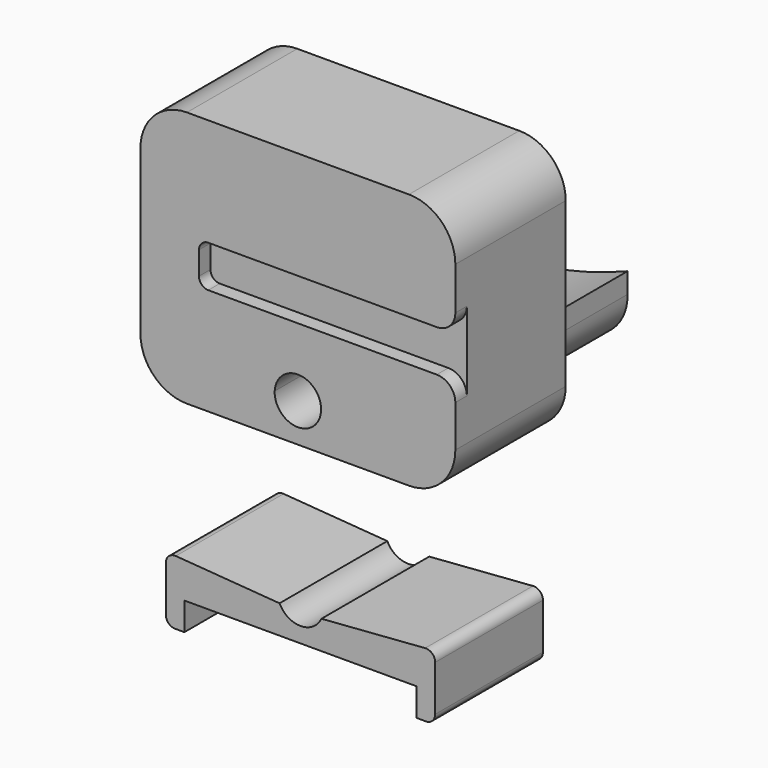
from build123d import *
from build123d import SkipClean  # not in build123d's __all__

# Parameters (mm, degrees)
F1_DEPTH  = 14.85
F2_DEPTH  = 13.3
F3_START  = 4
F3_DEPTH  = 9.3
F4_DEPTH  = 4
F5_START  = 4
F5_DEPTH  = 10.85
F6_R      = 1
F8_DEPTH  = 14.5
F9_DEPTH  = 3
F10_DEPTH = 2
F12_DEPTH = 14.5


with BuildPart() as f1:
    # F0 (on Front) → F1 (new body)
    with BuildSketch(Plane.XZ):
        with BuildLine():
            Line((11.95, 13.8), (-11.95, 13.8))
            ThreePointArc((-11.95, 13.8), (-15.4855339059, 12.3355339059), (-16.95, 8.8))
            Line((-16.95, 8.8), (-16.95, -5.8895261027))
            ThreePointArc((-16.95, -5.8895261027), (-9.8804541895, -8.3334638669), (-2.4972846772, -9.5335129141))
            ThreePointArc((-2.4972846772, -9.5335129141), (0.0448690015, -7.1504026779), (2.4998564985, -9.6232140564))
            ThreePointArc((2.4998564985, -9.6232140564), (9.8559923461, -8.7028657635), (16.95, -6.55))
            Line((16.95, -6.55), (16.95, -4.3))
            ThreePointArc((16.95, -4.3), (16.3642135624, -2.8857864376), (14.95, -2.3))
            Line((14.95, -2.3), (4.4395945761, -2.3))
            ThreePointArc((4.4395945761, -2.3), (0, -5), (-4.4395945761, -2.3))
            Line((-4.4395945761, -2.3), (-10.65, -2.3))
            Line((-10.65, -2.3), (-10.65, 2.2))
            Line((-10.65, 2.2), (-4.4899888641, 2.2))
            ThreePointArc((-4.4899888641, 2.2), (0, 5), (4.4899888641, 2.2))
            Line((4.4899888641, 2.2), (14.95, 2.2))
            ThreePointArc((14.95, 2.2), (16.3642135624, 2.7857864376), (16.95, 4.2))
            Line((16.95, 4.2), (16.95, 8.8))
            ThreePointArc((16.95, 8.8), (15.4855339059, 12.3355339059), (11.95, 13.8))
        make_face()
        with BuildLine():
            ThreePointArc((-2.4972846772, -9.5335129141), (-9.8804541895, -8.3334638669), (-16.95, -5.8895261027))
            Line((-16.95, -5.8895261027), (-16.95, -8.8))
            ThreePointArc((-16.95, -8.8), (-15.4855339059, -12.3355339059), (-11.95, -13.8))
            Line((-11.95, -13.8), (11.95, -13.8))
            ThreePointArc((11.95, -13.8), (15.4855339059, -12.3355339059), (16.95, -8.8))
            Line((16.95, -8.8), (16.95, -6.55))
            ThreePointArc((16.95, -6.55), (9.8559923461, -8.7028657635), (2.4998564985, -9.6232140564))
            ThreePointArc((2.4998564985, -9.6232140564), (2.4999641244, -9.636606836), (2.5, -9.65))
            ThreePointArc((2.5, -9.65), (-0.0582593644, -12.1493210771), (-2.4972846772, -9.5335129141))
        make_face()
    extrude(amount=F1_DEPTH)

    # F0 (on Front) → F2 (join)
    with BuildSketch(Plane.XZ):
        with BuildLine():
            ThreePointArc((-4.4395945761, -2.3), (-4.9996865006, -0.0559901426), (-4.4899888641, 2.2))
            Line((-4.4899888641, 2.2), (-10.65, 2.2))
            Line((-10.65, 2.2), (-10.65, -2.3))
            Line((-10.65, -2.3), (-4.4395945761, -2.3))
        make_face()
        with BuildLine():
            ThreePointArc((5, 0), (4.8708286934, 1.1291713066), (4.4899888641, 2.2))
            Line((4.4899888641, 2.2), (-4.4899888641, 2.2))
            ThreePointArc((-4.4899888641, 2.2), (-4.9996865006, -0.0559901426), (-4.4395945761, -2.3))
            Line((-4.4395945761, -2.3), (4.4395945761, -2.3))
            ThreePointArc((4.4395945761, -2.3), (4.8578788005, -1.1836441863), (5, 0))
        make_face()
        with BuildLine():
            Line((16.95, 2.2), (16.95, 4.2))
            ThreePointArc((16.95, 4.2), (16.3642135624, 2.7857864376), (14.95, 2.2))
            Line((14.95, 2.2), (4.4899888641, 2.2))
            ThreePointArc((4.4899888641, 2.2), (4.8708286934, 1.1291713066), (5, 0))
            ThreePointArc((5, 0), (4.8578788005, -1.1836441863), (4.4395945761, -2.3))
            Line((4.4395945761, -2.3), (14.95, -2.3))
            ThreePointArc((14.95, -2.3), (16.3642135624, -2.8857864376), (16.95, -4.3))
            Line((16.95, -4.3), (16.95, -2.3))
            Line((16.95, -2.3), (16.95, 2.2))
        make_face()
    extrude(amount=F2_DEPTH)

    # F0 (on Front) → F3 (join)
    with BuildSketch(Plane.XZ.offset(F3_START)):
        with BuildLine():
            Line((-4.4899888641, 2.2), (4.4899888641, 2.2))
            ThreePointArc((4.4899888641, 2.2), (0, 5), (-4.4899888641, 2.2))
        make_face()
        with BuildLine():
            Line((4.4395945761, -2.3), (-4.4395945761, -2.3))
            ThreePointArc((-4.4395945761, -2.3), (0, -5), (4.4395945761, -2.3))
        make_face()
        with BuildLine():
            ThreePointArc((5, 0), (4.8708286934, 1.1291713066), (4.4899888641, 2.2))
            Line((4.4899888641, 2.2), (-4.4899888641, 2.2))
            ThreePointArc((-4.4899888641, 2.2), (-4.9996865006, -0.0559901426), (-4.4395945761, -2.3))
            Line((-4.4395945761, -2.3), (4.4395945761, -2.3))
            ThreePointArc((4.4395945761, -2.3), (4.8578788005, -1.1836441863), (5, 0))
        make_face()
    extrude(amount=F3_DEPTH)

    # F0 (on Front) → F4 (cut)
    with BuildSketch(Plane.XZ):
        with BuildLine():
            ThreePointArc((5, 0), (4.8708286934, 1.1291713066), (4.4899888641, 2.2))
            Line((4.4899888641, 2.2), (-4.4899888641, 2.2))
            ThreePointArc((-4.4899888641, 2.2), (-4.9996865006, -0.0559901426), (-4.4395945761, -2.3))
            Line((-4.4395945761, -2.3), (4.4395945761, -2.3))
            ThreePointArc((4.4395945761, -2.3), (4.8578788005, -1.1836441863), (5, 0))
        make_face()
    with SkipClean():  # cleaning this boolean's faces spoils the solid; the shape is the same uncleaned
        extrude(amount=F4_DEPTH, mode=Mode.SUBTRACT)

    # F0 (on Front) → F5 (join)
    with BuildSketch(Plane.XZ.offset(F5_START)):
        with BuildLine():
            Line((-4.4899888641, 2.2), (4.4899888641, 2.2))
            ThreePointArc((4.4899888641, 2.2), (0, 5), (-4.4899888641, 2.2))
        make_face()
        with BuildLine():
            Line((4.4395945761, -2.3), (-4.4395945761, -2.3))
            ThreePointArc((-4.4395945761, -2.3), (0, -5), (4.4395945761, -2.3))
        make_face()
    with SkipClean():  # cleaning this boolean's faces spoils the solid; the shape is the same uncleaned
        extrude(amount=F5_DEPTH)

    # F6
    f6_edges = [f1.edges().sort_by_distance(p)[0] for p in [
        (-10.65, -14.075, 2.2),
        (-10.65, -14.075, -2.3),
    ]]
    fillet(f6_edges, radius=F6_R)


with BuildPart() as f8:
    # F7 (on Front) → F8 (new body)
    with BuildSketch(Plane.XZ):
        with BuildLine():
            ThreePointArc((-21.773402003, -7.6886942186), (-20.308935909, -11.2242281245), (-16.773402003, -12.6886942186))
            Line((-16.773402003, -12.6886942186), (7.0104826284, -12.6886942186))
            ThreePointArc((7.0104826284, -12.6886942186), (10.5825591861, -11.187303809), (12.0094031494, -7.584801845))
            Line((12.0094031494, -7.584801845), (12.0094031494, -5.3867480318))
            ThreePointArc((12.0094031494, -5.3867480318), (4.9971655581, -7.5221412361), (-2.2736510197, -8.4530582387))
            ThreePointArc((-2.2736510197, -8.4530582387), (-2.273464258, -8.4708757937), (-2.273402003, -8.4886942186))
            ThreePointArc((-2.273402003, -8.4886942186), (-4.8801320097, -11.0380631025), (-7.3708778511, -8.3752622863))
            ThreePointArc((-7.3708778511, -8.3752622863), (-14.7262981055, -7.1939892841), (-21.773402003, -4.7782203213))
            Line((-21.773402003, -4.7782203213), (-21.773402003, -7.6886942186))
        make_face()
    extrude(amount=-F8_DEPTH)

    # F7 (on Front) → F9 (join)
    with BuildSketch(Plane.XZ):
        with BuildLine():
            Line((-21.773402003, 3.4613057814), (-21.773402003, -4.7782203213))
            ThreePointArc((-21.773402003, -4.7782203213), (-14.7262981055, -7.1939892841), (-7.3708778511, -8.3752622863))
            ThreePointArc((-7.3708778511, -8.3752622863), (-4.7844873963, -5.9389911666), (-2.2736510197, -8.4530582387))
            ThreePointArc((-2.2736510197, -8.4530582387), (4.9971655581, -7.5221412361), (12.0094031494, -5.3867480318))
            Line((12.0094031494, -5.3867480318), (12.0094031494, -3.1886942186))
            ThreePointArc((12.0094031494, -3.1886942186), (11.4236167118, -1.7744806562), (10.0094031494, -1.1886942186))
            Line((10.0094031494, -1.1886942186), (-15.5905968506, -1.1886942186))
            Line((-15.5905968506, -1.1886942186), (-15.5905968506, 3.6113057814))
            Line((-15.5905968506, 3.6113057814), (10.0150360819, 3.6113057814))
            ThreePointArc((10.0150360819, 3.6113057814), (11.3751831327, 4.1450179515), (12.0094031494, 5.4613057814))
            Line((12.0094031494, 5.4613057814), (-19.773402003, 5.4613057814))
            ThreePointArc((-19.773402003, 5.4613057814), (-21.1876155654, 4.8755193438), (-21.773402003, 3.4613057814))
        make_face()
        with BuildLine():
            ThreePointArc((10.0094031494, -1.1886942186), (11.4236167118, -1.7744806562), (12.0094031494, -3.1886942186))
            Line((12.0094031494, -3.1886942186), (12.0094031494, -1.1886942186))
            Line((12.0094031494, -1.1886942186), (12.0094031494, 3.3113057814))
            Line((12.0094031494, 3.3113057814), (12.0094031494, 5.4613057814))
            ThreePointArc((12.0094031494, 5.4613057814), (11.3751831327, 4.1450179515), (10.0150360819, 3.6113057814))
            Line((10.0150360819, 3.6113057814), (-15.5905968506, 3.6113057814))
            Line((-15.5905968506, 3.6113057814), (-15.5905968506, -1.1886942186))
            Line((-15.5905968506, -1.1886942186), (10.0094031494, -1.1886942186))
        make_face()
    extrude(amount=-F9_DEPTH)

    # F7 (on Front) → F10 (cut)
    with BuildSketch(Plane.XZ):
        with BuildLine():
            ThreePointArc((10.0094031494, -1.1886942186), (11.4236167118, -1.7744806562), (12.0094031494, -3.1886942186))
            Line((12.0094031494, -3.1886942186), (12.0094031494, -1.1886942186))
            Line((12.0094031494, -1.1886942186), (12.0094031494, 3.3113057814))
            Line((12.0094031494, 3.3113057814), (12.0094031494, 5.4613057814))
            ThreePointArc((12.0094031494, 5.4613057814), (11.3751831327, 4.1450179515), (10.0150360819, 3.6113057814))
            Line((10.0150360819, 3.6113057814), (-15.5905968506, 3.6113057814))
            Line((-15.5905968506, 3.6113057814), (-15.5905968506, -1.1886942186))
            Line((-15.5905968506, -1.1886942186), (10.0094031494, -1.1886942186))
        make_face()
    extrude(amount=-F10_DEPTH, mode=Mode.SUBTRACT)


with BuildPart() as f12:
    # F11 (on Front) → F12 (new body)
    with BuildSketch(Plane.XZ):
        with BuildLine():
            Line((-12.5, -32.7800722122), (0, -32.7800722122))
            Line((0, -32.7800722122), (12.5, -32.7800722122))
            Line((12.5, -32.7800722122), (12.5, -35.7800722122))
            Line((12.5, -35.7800722122), (13.5, -35.7800722122))
            ThreePointArc((13.5, -35.7800722122), (14.2071067812, -35.4871789934), (14.5, -34.7800722122))
            Line((14.5, -34.7800722122), (14.5, -29.8588076797))
            ThreePointArc((14.5, -29.8588076797), (14.1798364834, -29.1254439529), (13.4243552884, -28.8616728455))
            Line((13.4243552884, -28.8616728455), (2.255203111, -29.7089878383))
            ThreePointArc((2.255203111, -29.7089878383), (0, -31.1300722122), (-2.255203111, -29.7089878383))
            Line((-2.255203111, -29.7089878383), (-13.4243552884, -28.8616728455))
            ThreePointArc((-13.4243552884, -28.8616728455), (-14.1798364834, -29.1254439529), (-14.5, -29.8588076797))
            Line((-14.5, -29.8588076797), (-14.5, -34.7800722122))
            ThreePointArc((-14.5, -34.7800722122), (-14.2071067812, -35.4871789934), (-13.5, -35.7800722122))
            Line((-13.5, -35.7800722122), (-12.5, -35.7800722122))
            Line((-12.5, -35.7800722122), (-12.5, -32.7800722122))
        make_face()
    extrude(amount=F12_DEPTH)


solid = Compound([f1.part, f8.part, f12.part])
